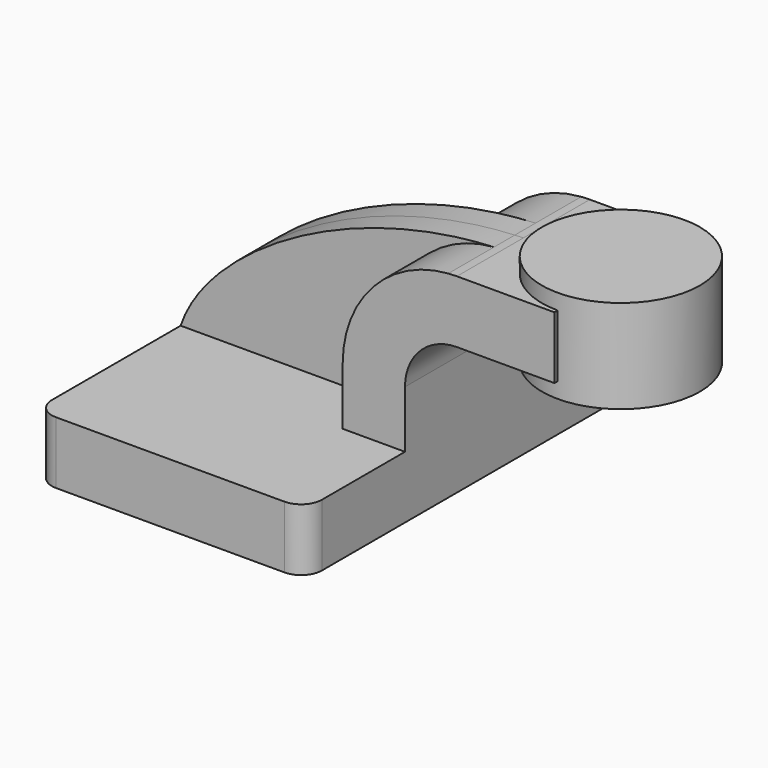
from build123d import *

# Parameters (mm, degrees)
F1_DEPTH = 63.5
F0_W     = 26.6420548012
F0_H     = 19.05
F2_DEPTH = 25.4
F3_DEPTH = 7.9375
F5_R     = 6.35


# Not quite as in the source:
# - a feature of the source that left no trace in its solid (it failed there, or was rolled back) is left out


with BuildPart() as f1:
    # F0 (on Front) → F1 (new body, symmetric)
    with BuildSketch(Plane.XZ):
        Polygon((-41.275, 9.525), (-41.275, -9.525), (41.275, -9.525), (41.275, 9.525), (22.225, 9.525), align=None)
    extrude(amount=F1_DEPTH, both=True)

    # F0 (on Front) → F2 (join, symmetric)
    with BuildSketch(Plane.XZ):
        with BuildLine():
            Line((22.225, 9.525), (41.275, 9.525))
            Line((41.275, 9.525), (41.275, 27.0002))
            ThreePointArc((41.275, 27.0002), (45.9246798487, 38.2255201513), (57.15, 42.8752))
            Line((57.15, 42.8752), (60.325, 42.8752))
            Line((60.325, 42.8752), (60.325, 61.9252))
            Line((60.325, 61.9252), (57.15, 61.9252))
            add(Edge.make_bspline(
                [(54.5213953348, 61.8261395066), (55.3958874756, 61.867746875), (56.2721525992, 61.9008262266), (57.15, 61.9252)],
                knots=[109.4468822065, 109.4468822065, 109.4468822065, 109.4468822065, 111.5045361635, 111.5045361635, 111.5045361635, 111.5045361635], degree=3))
            ThreePointArc((54.5213953348, 61.8261395066), (31.5418016747, 50.7483747411), (22.225, 27.0002))
            Line((22.225, 27.0002), (22.225, 9.525))
        make_face()
        with Locations((73.6460274006, 52.4002)):
            Rectangle(F0_W, F0_H)
    extrude(amount=F2_DEPTH, both=True)

    # F0 (on Front) → F3 (join, symmetric)
    with BuildSketch(Plane.XZ):
        with BuildLine():
            add(Edge.make_bspline(
                [(-41.275, 9.525), (-33.4912011652, 33.272556952), (8.0070443726, 59.6130381539), (54.5213953348, 61.8261395066)],
                knots=[0, 0, 0, 0, 109.4468822065, 109.4468822065, 109.4468822065, 109.4468822065], degree=3))
            Line((-41.275, 9.525), (22.225, 9.525))
            Line((22.225, 9.525), (22.225, 27.0002))
            ThreePointArc((22.225, 27.0002), (31.5418016747, 50.7483747411), (54.5213953348, 61.8261395066))
        make_face()
    extrude(amount=F3_DEPTH, both=True)

    # F0 (on Front) → F4 (revolve)
    with BuildSketch(Plane.XZ):
        Polygon((86.9670548012, 66.675), (86.9670548012, 61.9252), (86.9670548012, 42.8752), (86.9670548012, 38.1), (111.125, 38.1), (111.125, 66.675), align=None)
    revolve(axis=Axis((86.9670548012, 0, 52.3875), (0, 0, 1)))

    # F5
    f5_edges = [f1.edges().sort_by_distance(p)[0] for p in [
        (-41.275, -63.5, 0),
        (41.275, -63.5, 0),
        (41.275, 63.5, 0),
        (-41.275, 63.5, 0),
    ]]
    fillet(f5_edges, radius=F5_R)


solid = f1.part
